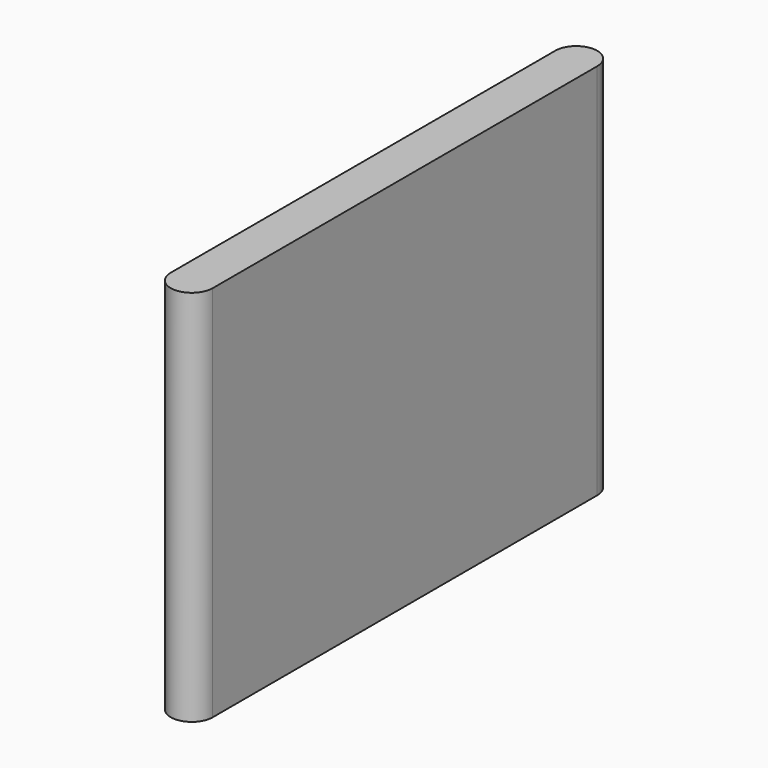
from build123d import *

# Parameters (mm, degrees)
F1_DEPTH = 18


# Not quite as in the source:
# - ends of sketch curves that miss each other by under 0.0002 mm in the source are joined


with BuildPart() as f1:
    # F0 (on Top) → F1 (new body, symmetric)
    with BuildSketch(Plane.XY):
        with BuildLine():
            Line((1.9999976953, -23.3999992664), (1.9999976953, 22.4000007336))
            ThreePointArc((1.9999976953, 22.4000007336), (2.3047e-06, 24.3999961241), (-1.9999930858, 22.4000007336))
            Line((-1.9999930858, 22.4000007336), (-1.9999976953, -23.3999992664))
            ThreePointArc((-1.9999976953, -23.3999992664), (-2.3047e-06, -25.3999992664), (1.9999976953, -23.3999992664))
        make_face()
    extrude(amount=F1_DEPTH, both=True)


solid = f1.part
